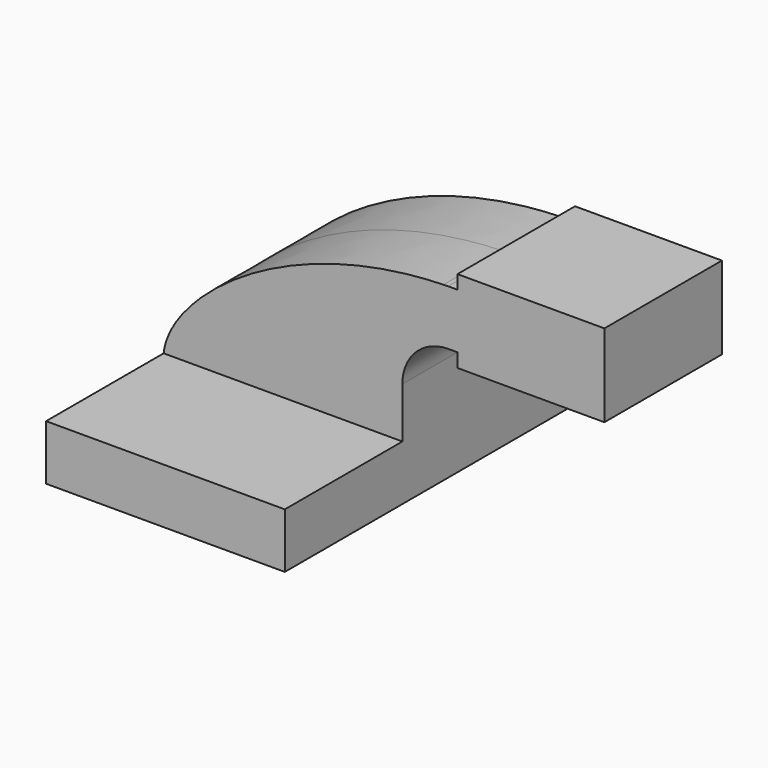
from build123d import *

# Parameters (mm, degrees)
F0_W     = 25.4
F0_H     = 19.05
F1_DEPTH = 25.4
F2_DEPTH = 12.7
F3_DEPTH = 63.5


# Not quite as in the source:
# - a feature of the source that left no trace in its solid (it failed there, or was rolled back) is left out


with BuildPart() as f1:
    # F0 (on Front) → F1 (new body, symmetric)
    with BuildSketch(Plane.XZ):
        with BuildLine():
            add(Edge.make_bspline(
                [(-41.275, 9.525), (-39.3446406739, 28.5086459931), (-0.7471661584, 60.2765032574), (55.5187541124, 61.8870838083)],
                knots=[0, 0, 0, 0, 110.4404580892, 110.4404580892, 110.4404580892, 110.4404580892], degree=3))
            Line((-41.275, 9.525), (22.225, 9.525))
            Line((22.225, 9.525), (22.225, 27.0002))
            ThreePointArc((22.225, 27.0002), (31.8841447045, 51.1122754227), (55.5187541124, 61.8870838083))
        make_face()
        with BuildLine():
            Line((22.225, 9.525), (41.275, 9.525))
            Line((41.275, 9.525), (41.275, 27.0002))
            ThreePointArc((41.275, 27.0002), (45.9246798487, 38.2255201513), (57.15, 42.8752))
            Line((57.15, 42.8752), (60.325, 42.8752))
            Line((60.325, 42.8752), (60.325, 61.9252))
            Line((60.325, 61.9252), (57.15, 61.9252))
            add(Edge.make_bspline(
                [(55.5187541124, 61.8870838083), (56.0608682355, 61.9026015224), (56.6046225289, 61.915319722), (57.15, 61.9252)],
                knots=[110.4404580892, 110.4404580892, 110.4404580892, 110.4404580892, 111.5045361635, 111.5045361635, 111.5045361635, 111.5045361635], degree=3))
            ThreePointArc((55.5187541124, 61.8870838083), (31.8841447045, 51.1122754227), (22.225, 27.0002))
            Line((22.225, 27.0002), (22.225, 9.525))
        make_face()
        with Locations((73.025, 52.4002)):
            Rectangle(F0_W, F0_H)
        Polygon((60.325, 66.675), (60.325, 61.9252), (85.725, 61.9252), (85.725, 42.8752), (60.325, 42.8752), (60.325, 38.1), (111.125, 38.1), (111.125, 66.675), align=None)
    extrude(amount=F1_DEPTH, both=True)

    # F0 (on Front) → F2 (join, symmetric)
    with BuildSketch(Plane.XZ):
        Polygon((-41.275, 9.525), (-41.275, -9.525), (41.275, -9.525), (41.275, 9.525), (22.225, 9.525), align=None)
        with BuildLine():
            add(Edge.make_bspline(
                [(-41.275, 9.525), (-39.3446406739, 28.5086459931), (-0.7471661584, 60.2765032574), (55.5187541124, 61.8870838083)],
                knots=[0, 0, 0, 0, 110.4404580892, 110.4404580892, 110.4404580892, 110.4404580892], degree=3))
            Line((-41.275, 9.525), (22.225, 9.525))
            Line((22.225, 9.525), (22.225, 27.0002))
            ThreePointArc((22.225, 27.0002), (31.8841447045, 51.1122754227), (55.5187541124, 61.8870838083))
        make_face()
        with BuildLine():
            Line((22.225, 9.525), (41.275, 9.525))
            Line((41.275, 9.525), (41.275, 27.0002))
            ThreePointArc((41.275, 27.0002), (45.9246798487, 38.2255201513), (57.15, 42.8752))
            Line((57.15, 42.8752), (60.325, 42.8752))
            Line((60.325, 42.8752), (60.325, 61.9252))
            Line((60.325, 61.9252), (57.15, 61.9252))
            add(Edge.make_bspline(
                [(55.5187541124, 61.8870838083), (56.0608682355, 61.9026015224), (56.6046225289, 61.915319722), (57.15, 61.9252)],
                knots=[110.4404580892, 110.4404580892, 110.4404580892, 110.4404580892, 111.5045361635, 111.5045361635, 111.5045361635, 111.5045361635], degree=3))
            ThreePointArc((55.5187541124, 61.8870838083), (31.8841447045, 51.1122754227), (22.225, 27.0002))
            Line((22.225, 27.0002), (22.225, 9.525))
        make_face()
        with Locations((73.025, 52.4002)):
            Rectangle(F0_W, F0_H)
        Polygon((60.325, 66.675), (60.325, 61.9252), (85.725, 61.9252), (85.725, 42.8752), (60.325, 42.8752), (60.325, 38.1), (111.125, 38.1), (111.125, 66.675), align=None)
    extrude(amount=F2_DEPTH, both=True)

    # F3 (add, symmetric): a face of the model
    f3_faces = [f1.faces().sort_by_distance(p)[0] for p in [
        (0, -12.7, 0),
    ]]
    extrude(f3_faces, amount=F3_DEPTH, both=True)


solid = f1.part
